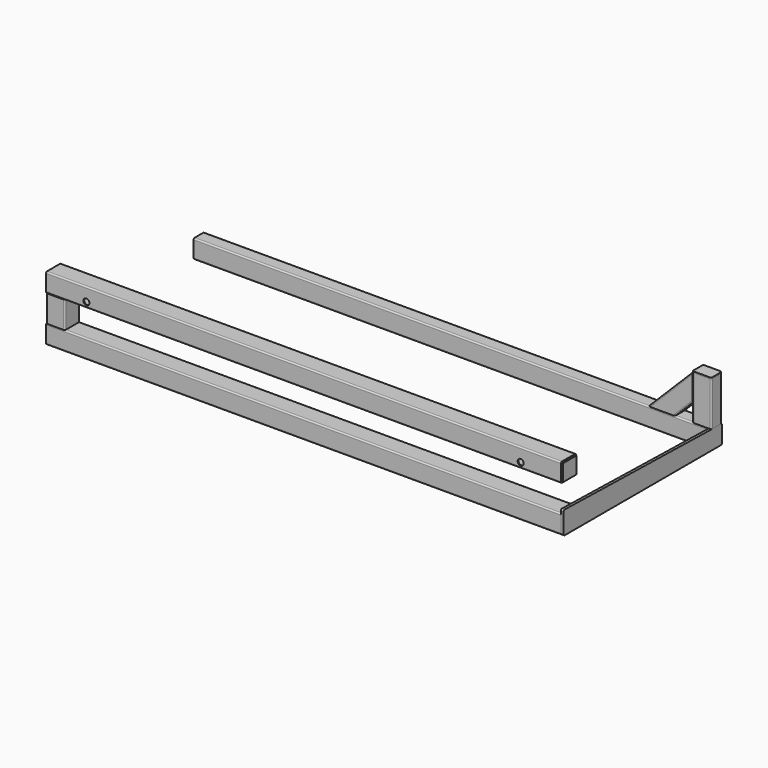
from build123d import *

# Parameters (mm, degrees)
F1_DEPTH  = 2446.528
F3_DEPTH  = 254
F5_DEPTH  = 2446.528
F7_DEPTH  = 25.4
F9_DEPTH  = 2446.528
F11_DEPTH = 419.1
F13_DEPTH = 127
F14_R     = 12.7
F15_T     = -9.525
F17_DEPTH = 12.7
F19_DEPTH = 12.7
F20_R     = 9.652
F21_DEPTH = 19.05
F23_DEPTH = 19.05
F24_R     = 28.575
F25_DEPTH = 1879.601


with BuildPart() as f1:
    # F0 (on Right) → F1 (new body, symmetric)
    with BuildSketch(Plane.YZ):
        with BuildLine():
            ThreePointArc((0, 12.7), (3.7197438789, 3.7197438789), (12.7, 0))
            Line((12.7, 0), (165.1, 0))
            ThreePointArc((165.1, 0), (174.0802561211, 3.7197438789), (177.8, 12.7))
            Line((177.8, 12.7), (177.8, 165.1))
            ThreePointArc((177.8, 165.1), (174.0802561211, 174.0802561211), (165.1, 177.8))
            Line((165.1, 177.8), (12.7, 177.8))
            ThreePointArc((12.7, 177.8), (3.7197438789, 174.0802561211), (0, 165.1))
            Line((0, 165.1), (0, 12.7))
        make_face()
        with BuildLine():
            ThreePointArc((9.525, 165.1), (10.4549359697, 167.3450640303), (12.7, 168.275))
            Line((12.7, 168.275), (165.1, 168.275))
            ThreePointArc((165.1, 168.275), (167.3450640303, 167.3450640303), (168.275, 165.1))
            Line((168.275, 165.1), (168.275, 12.7))
            ThreePointArc((168.275, 12.7), (167.3450640303, 10.4549359697), (165.1, 9.525))
            Line((165.1, 9.525), (12.7, 9.525))
            ThreePointArc((12.7, 9.525), (10.4549359697, 10.4549359697), (9.525, 12.7))
            Line((9.525, 12.7), (9.525, 165.1))
        make_face(mode=Mode.SUBTRACT)
    extrude(amount=F1_DEPTH, both=True)


with BuildPart() as f3:
    # F2 (on face) → F3 (new body)
    with BuildSketch(Plane.XY.offset(177.8)):
        with BuildLine():
            ThreePointArc((-2446.528, 12.7), (-2442.8082561211, 3.7197438789), (-2433.828, 0))
            Line((-2433.828, 0), (-2281.428, 0))
            ThreePointArc((-2281.428, 0), (-2272.4477438789, 3.7197438789), (-2268.728, 12.7))
            Line((-2268.728, 12.7), (-2268.728, 165.1))
            ThreePointArc((-2268.728, 165.1), (-2272.4477438789, 174.0802561211), (-2281.428, 177.8))
            Line((-2281.428, 177.8), (-2433.828, 177.8))
            ThreePointArc((-2433.828, 177.8), (-2442.8082561211, 174.0802561211), (-2446.528, 165.1))
            Line((-2446.528, 165.1), (-2446.528, 12.7))
        make_face()
        with BuildLine():
            ThreePointArc((-2437.003, 165.1), (-2436.0730640303, 167.3450640303), (-2433.828, 168.275))
            Line((-2433.828, 168.275), (-2281.428, 168.275))
            ThreePointArc((-2281.428, 168.275), (-2279.1829359697, 167.3450640303), (-2278.253, 165.1))
            Line((-2278.253, 165.1), (-2278.253, 12.7))
            ThreePointArc((-2278.253, 12.7), (-2279.1829359697, 10.4549359697), (-2281.428, 9.525))
            Line((-2281.428, 9.525), (-2433.828, 9.525))
            ThreePointArc((-2433.828, 9.525), (-2436.0730640303, 10.4549359697), (-2437.003, 12.7))
            Line((-2437.003, 12.7), (-2437.003, 165.1))
        make_face(mode=Mode.SUBTRACT)
    extrude(amount=F3_DEPTH)


with BuildPart() as f5:
    # F4 (on Right) → F5 (new body, symmetric)
    with BuildSketch(Plane.YZ):
        with BuildLine():
            ThreePointArc((0, 444.5), (3.7197438789, 435.5197438789), (12.7, 431.8))
            Line((12.7, 431.8), (165.1, 431.8))
            ThreePointArc((165.1, 431.8), (174.0802561211, 435.5197438789), (177.8, 444.5))
            Line((177.8, 444.5), (177.8, 596.9))
            ThreePointArc((177.8, 596.9), (174.0802561211, 605.8802561211), (165.1, 609.6))
            Line((165.1, 609.6), (12.7, 609.6))
            ThreePointArc((12.7, 609.6), (3.7197438789, 605.8802561211), (0, 596.9))
            Line((0, 596.9), (0, 444.5))
        make_face()
        with BuildLine():
            ThreePointArc((9.525, 596.9), (10.4549359697, 599.1450640303), (12.7, 600.075))
            Line((12.7, 600.075), (165.1, 600.075))
            ThreePointArc((165.1, 600.075), (167.3450640303, 599.1450640303), (168.275, 596.9))
            Line((168.275, 596.9), (168.275, 444.5))
            ThreePointArc((168.275, 444.5), (167.3450640303, 442.2549359697), (165.1, 441.325))
            Line((165.1, 441.325), (12.7, 441.325))
            ThreePointArc((12.7, 441.325), (10.4549359697, 442.2549359697), (9.525, 444.5))
            Line((9.525, 444.5), (9.525, 596.9))
        make_face(mode=Mode.SUBTRACT)
    extrude(amount=F5_DEPTH, both=True)

    # F24 (on face) → F25 (cut, through all)
    with BuildSketch(Plane.XZ):
        with Locations((-2063.2928, 482.6)):
            Circle(F24_R)
        with Locations((2063.2928, 482.6)):
            Circle(F24_R)
    extrude(amount=-F25_DEPTH, mode=Mode.SUBTRACT)


with BuildPart() as f7:
    # F6 (on face) → F7 (new body)
    with BuildSketch(Plane.YZ.offset(2446.528)):
        with BuildLine():
            ThreePointArc((0, 12.7), (3.7197438789, 3.7197438789), (12.7, 0))
            Line((12.7, 0), (1866.9, 0))
            ThreePointArc((1866.9, 0), (1875.8802561211, 3.7197438789), (1879.6, 12.7))
            Line((1879.6, 12.7), (1879.6, 165.1))
            ThreePointArc((1879.6, 165.1), (1875.8802561211, 174.0802561211), (1866.9, 177.8))
            Line((1866.9, 177.8), (1739.9, 177.8))
            Line((1739.9, 177.8), (12.9801243347, 215.9))
            ThreePointArc((12.9801243347, 215.9), (3.8193350207, 212.2818445763), (0, 203.2030897319))
            Line((0, 203.2030897319), (0, 12.7))
        make_face()
    extrude(amount=F7_DEPTH)


with BuildPart() as f9:
    # F8 (on Right) → F9 (new body, symmetric)
    with BuildSketch(Plane.YZ):
        with BuildLine():
            ThreePointArc((1752.6, 12.7), (1756.3197438789, 3.7197438789), (1765.3, 0))
            Line((1765.3, 0), (1866.9, 0))
            ThreePointArc((1866.9, 0), (1875.8802561211, 3.7197438789), (1879.6, 12.7))
            Line((1879.6, 12.7), (1879.6, 165.1))
            ThreePointArc((1879.6, 165.1), (1875.8802561211, 174.0802561211), (1866.9, 177.8))
            Line((1866.9, 177.8), (1765.3, 177.8))
            ThreePointArc((1765.3, 177.8), (1756.3197438789, 174.0802561211), (1752.6, 165.1))
            Line((1752.6, 165.1), (1752.6, 12.7))
        make_face()
        with BuildLine():
            ThreePointArc((1762.125, 165.1), (1763.0549359697, 167.3450640303), (1765.3, 168.275))
            Line((1765.3, 168.275), (1866.9, 168.275))
            ThreePointArc((1866.9, 168.275), (1869.1450640303, 167.3450640303), (1870.075, 165.1))
            Line((1870.075, 165.1), (1870.075, 12.7))
            ThreePointArc((1870.075, 12.7), (1869.1450640303, 10.4549359697), (1866.9, 9.525))
            Line((1866.9, 9.525), (1765.3, 9.525))
            ThreePointArc((1765.3, 9.525), (1763.0549359697, 10.4549359697), (1762.125, 12.7))
            Line((1762.125, 12.7), (1762.125, 165.1))
        make_face(mode=Mode.SUBTRACT)
    extrude(amount=F9_DEPTH, both=True)


with BuildPart() as f11:
    # F10 (on face) → F11 (new body)
    with BuildSketch(Plane.XY.offset(177.8)):
        with BuildLine():
            ThreePointArc((2294.128, 1765.3), (2297.8477438789, 1756.3197438789), (2306.828, 1752.6))
            Line((2306.828, 1752.6), (2459.228, 1752.6))
            ThreePointArc((2459.228, 1752.6), (2468.2082561211, 1756.3197438789), (2471.928, 1765.3))
            Line((2471.928, 1765.3), (2471.928, 1866.9))
            ThreePointArc((2471.928, 1866.9), (2468.2082561211, 1875.8802561211), (2459.228, 1879.6))
            Line((2459.228, 1879.6), (2306.828, 1879.6))
            ThreePointArc((2306.828, 1879.6), (2297.8477438789, 1875.8802561211), (2294.128, 1866.9))
            Line((2294.128, 1866.9), (2294.128, 1765.3))
        make_face()
        with BuildLine():
            ThreePointArc((2303.653, 1866.9), (2304.5829359697, 1869.1450640303), (2306.828, 1870.075))
            Line((2306.828, 1870.075), (2459.228, 1870.075))
            ThreePointArc((2459.228, 1870.075), (2461.4730640303, 1869.1450640303), (2462.403, 1866.9))
            Line((2462.403, 1866.9), (2462.403, 1765.3))
            ThreePointArc((2462.403, 1765.3), (2461.4730640303, 1763.0549359697), (2459.228, 1762.125))
            Line((2459.228, 1762.125), (2306.828, 1762.125))
            ThreePointArc((2306.828, 1762.125), (2304.5829359697, 1763.0549359697), (2303.653, 1765.3))
            Line((2303.653, 1765.3), (2303.653, 1866.9))
        make_face(mode=Mode.SUBTRACT)
    extrude(amount=F11_DEPTH)


with BuildPart() as f13:
    # F12 (on face) → F13 (new body, through all)
    with BuildSketch(Plane(origin=(0, 1879.6, 0), x_dir=(-1, 0, 0), z_dir=(0, 1, 0))):
        Polygon((-1875.028, 177.8), (-2294.128, 596.9), (-2294.128, 345.4528286101), (-2126.4751713899, 177.8), align=None)
    extrude(amount=-F13_DEPTH)

    # F14
    f14_edges = [f13.edges().sort_by_distance(p)[0] for p in [
        (2084.578, 1879.6, 387.35),
        (2210.301586, 1879.6, 261.626414),
        (2084.578, 1752.6, 387.35),
        (2210.301586, 1752.6, 261.626414),
    ]]
    fillet(f14_edges, radius=F14_R)

    # F15
    f15_openings = [f13.faces().sort_by_distance(p)[0] for p in [
        (2294.128, 1816.1, 471.176414),
        (2000.751586, 1816.1, 177.8),
    ]]
    offset(amount=F15_T, openings=f15_openings)


with BuildPart() as f17:
    # F16 (on face) → F17 (new body)
    with BuildSketch(Plane.XY.offset(596.9)):
        with BuildLine():
            ThreePointArc((2294.128, 1765.3), (2297.8477438789, 1756.3197438789), (2306.828, 1752.6))
            Line((2306.828, 1752.6), (2459.228, 1752.6))
            ThreePointArc((2459.228, 1752.6), (2468.2082561211, 1756.3197438789), (2471.928, 1765.3))
            Line((2471.928, 1765.3), (2471.928, 1866.9))
            ThreePointArc((2471.928, 1866.9), (2468.2082561211, 1875.8802561211), (2459.228, 1879.6))
            Line((2459.228, 1879.6), (2306.828, 1879.6))
            ThreePointArc((2306.828, 1879.6), (2297.8477438789, 1875.8802561211), (2294.128, 1866.9))
            Line((2294.128, 1866.9), (2294.128, 1765.3))
        make_face()
    extrude(amount=F17_DEPTH)


with BuildPart() as f19:
    # F18 (on face) → F19 (new body)
    with BuildSketch(Plane.YZ.offset(2446.528)):
        with BuildLine():
            Line((165.1, 600.075), (12.7, 600.075))
            ThreePointArc((12.7, 600.075), (10.4549359697, 599.1450640303), (9.525, 596.9))
            Line((9.525, 596.9), (9.525, 444.5))
            ThreePointArc((9.525, 444.5), (10.4549359697, 442.2549359697), (12.7, 441.325))
            Line((12.7, 441.325), (165.1, 441.325))
            ThreePointArc((165.1, 441.325), (167.3450640303, 442.2549359697), (168.275, 444.5))
            Line((168.275, 444.5), (168.275, 596.9))
            ThreePointArc((168.275, 596.9), (167.3450640303, 599.1450640303), (165.1, 600.075))
        make_face()
    extrude(amount=F19_DEPTH)


with BuildPart() as f21:
    # F20 (on face) → F21 (new body)
    with BuildSketch(Plane(origin=(0, 0, 0), x_dir=(1, 0, 0), z_dir=(0, 0, -1))):
        Polygon((2446.528, -1752.6), (2446.528, -177.8), (2319.528, -177.8), (2344.928, -685.8), (2344.928, -1447.8), (2319.528, -1752.6), align=None)
        with Locations((2377.948, -1057.275)):
            Circle(F20_R, mode=Mode.SUBTRACT)
        with Locations((2377.948, -873.125)):
            Circle(F20_R, mode=Mode.SUBTRACT)
    extrude(amount=F21_DEPTH)


with BuildPart() as f23:
    # F22 (on face) → F23 (new body)
    with BuildSketch(Plane.XZ.offset(-1752.6)):
        Polygon((2446.528, 0), (2446.528, 101.6), (2344.928, 0), align=None)
    extrude(amount=F23_DEPTH)


solid = Compound([f1.part, f3.part, f5.part, f7.part, f9.part, f11.part, f13.part, f17.part, f19.part, f21.part, f23.part])
